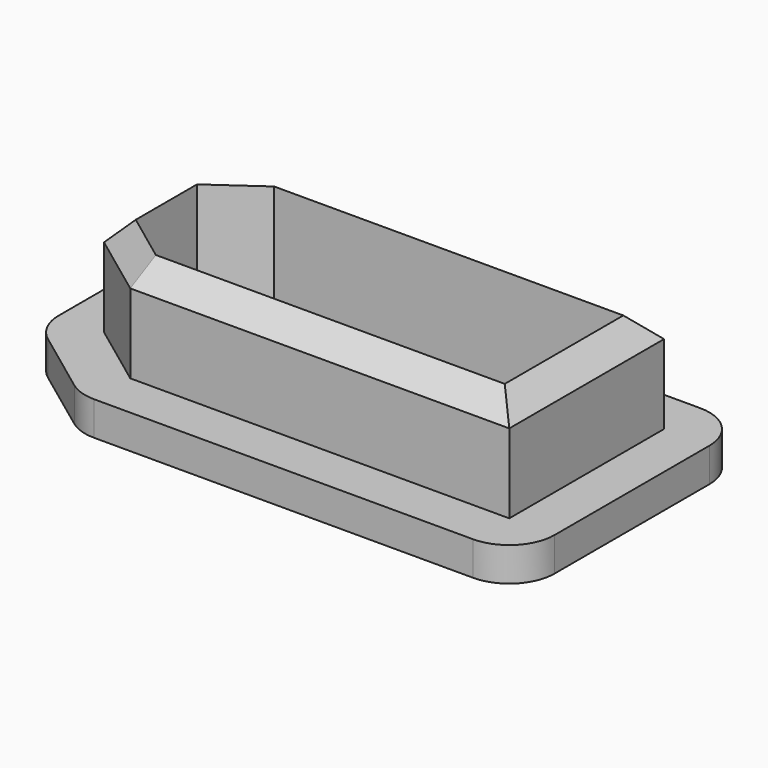
from build123d import *

# Parameters (mm, degrees)
F1_DEPTH     = 1.5
F2_DEPTH     = 6
F3_TEXT_SIZE = 6.4659554023
F4_DEPTH     = 0.75
F5_R         = 2
F6_SIZE      = 0.99999


# Not quite as in the source:
# - a fillet or chamfer is up to 0.001 mm smaller than in the source, because OpenCascade refuses the exact size
# - Text() gives the source's letters only with a copy of the font that has no kerning and outlines rounded to 1/6400 em; it was checked with that copy


with BuildPart() as f1:
    # F0 (on Top) → F1 (new body)
    with BuildSketch(Plane.XY):
        Polygon((2, -10.55), (2, 2), (-17.3862676957, 2), (-21.609642, -0.9897908086), (-21.609642, -7.4336311631), (-17.411145532, -10.55), align=None)
        Polygon((-16.75, 0), (0, 0), (0, -8.55), (-16.75, -8.55), (-19.609642, -6.427407), (-19.609642, -4.2258955), (-19.609642, -2.024384), align=None, mode=Mode.SUBTRACT)
        Polygon((0, -8.55), (0, 0), (-16.75, 0), (-19.609642, -2.024384), (-19.609642, -4.2258955), (-19.609642, -6.427407), (-16.75, -8.55), align=None)
        Polygon((-16.4318661521, -1), (-1, -1), (-1, -7.55), (-16.419427234, -7.55), (-18.609642, -5.9242949184), (-18.609642, -2.5416805957), align=None, mode=Mode.SUBTRACT)
        Polygon((-1, -7.55), (-1, -1), (-16.4318661521, -1), (-18.609642, -2.5416805957), (-18.609642, -5.9242949184), (-16.419427234, -7.55), align=None)
    extrude(amount=F1_DEPTH)

    # F0 (on Top) → F2 (join)
    with BuildSketch(Plane.XY):
        Polygon((0, -8.55), (0, 0), (-16.75, 0), (-19.609642, -2.024384), (-19.609642, -4.2258955), (-19.609642, -6.427407), (-16.75, -8.55), align=None)
        Polygon((-16.4318661521, -1), (-1, -1), (-1, -7.55), (-16.419427234, -7.55), (-18.609642, -5.9242949184), (-18.609642, -2.5416805957), align=None, mode=Mode.SUBTRACT)
    extrude(amount=F2_DEPTH)

    # F3 (on face) → F4 (cut)
    with BuildSketch(Plane(origin=(0, 0, 0), x_dir=(1, 0, 0), z_dir=(0, 0, -1))):
        with Locations((-15.999914055, 2.1569977028)):
            Text('H-13', F3_TEXT_SIZE, font='Open Sans', font_style=FontStyle.BOLD, text_align=(TextAlign.LEFT, TextAlign.BOTTOM))
    extrude(amount=-F4_DEPTH, mode=Mode.SUBTRACT)

    # F5
    f5_edges = [f1.edges().sort_by_distance(p)[0] for p in [
        (2, 2, 0.75),
        (2, -10.55, 0.75),
        (-21.609642, -0.989791, 0.75),
        (-21.609642, -7.433631, 0.75),
        (-17.386268, 2, 0.75),
        (-17.411146, -10.55, 0.75),
    ]]
    fillet(f5_edges, radius=F5_R)

    # F6 (size 1 in the source; OpenCascade refuses exactly that, so slightly less here)
    f6_edges = [f1.edges().sort_by_distance(p)[0] for p in [
        (-8.375, -8.55, 6),
        (0, -4.275, 6),
        (-8.375, 0, 6),
        (-18.179821, -1.012192, 6),
        (-19.609642, -4.225895, 6),
        (-18.179821, -7.488703, 6),
    ]]
    chamfer(f6_edges, length=F6_SIZE)


solid = f1.part
